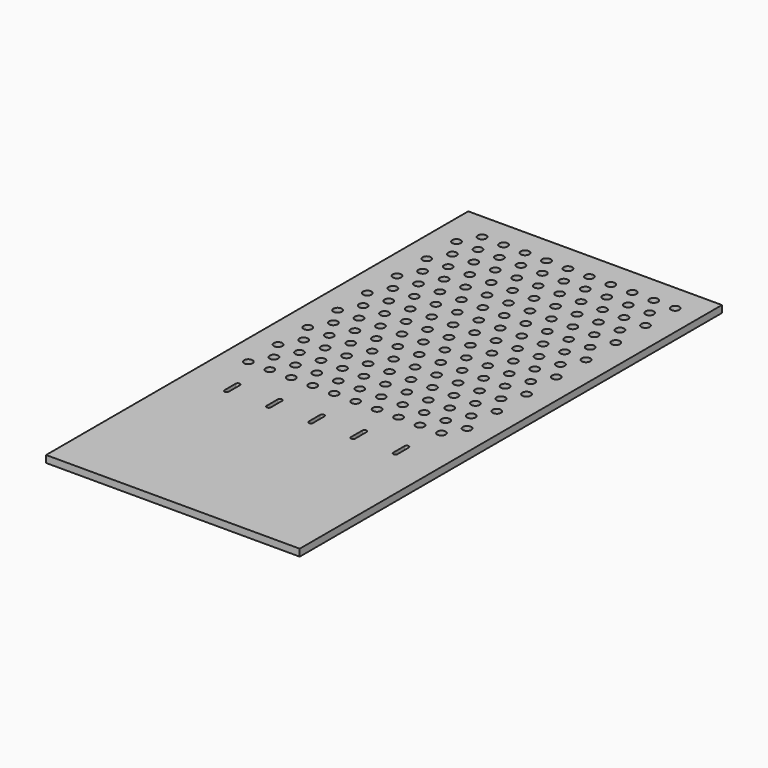
from build123d import *

# Parameters (mm, degrees)
F0_W     = 360.5
F0_H     = 750
F0_R     = 6
F1_DEPTH = 10
F3_DEPTH = 25


# Not quite as in the source:
# - a feature of the source that left no trace in its solid (it failed there, or was rolled back) is left out


with BuildPart() as f1:
    # F0 (on Top) → F1 (new body)
    with BuildSketch(Plane.XY):
        with Locations((145, 59.75)):
            Rectangle(F0_W, F0_H)
        Circle(F0_R, mode=Mode.SUBTRACT)
        with Locations((0, 52.828)):
            Circle(F0_R, mode=Mode.SUBTRACT)
        with Locations((30.5, 0)):
            Circle(F0_R, mode=Mode.SUBTRACT)
        with Locations((15.25, 26.4137748154)):
            Circle(F0_R, mode=Mode.SUBTRACT)
        with Locations((30.5, 52.828)):
            Circle(F0_R, mode=Mode.SUBTRACT)
        with Locations((45.75, 26.4137748154)):
            Circle(F0_R, mode=Mode.SUBTRACT)
        with Locations((61, 0)):
            Circle(F0_R, mode=Mode.SUBTRACT)
        with Locations((91.5, 0)):
            Circle(F0_R, mode=Mode.SUBTRACT)
        with Locations((76.25, 26.4137748154)):
            Circle(F0_R, mode=Mode.SUBTRACT)
        with Locations((61, 52.828)):
            Circle(F0_R, mode=Mode.SUBTRACT)
        with Locations((91.5, 52.828)):
            Circle(F0_R, mode=Mode.SUBTRACT)
        with Locations((122, 0)):
            Circle(F0_R, mode=Mode.SUBTRACT)
        with Locations((106.75, 26.4137748154)):
            Circle(F0_R, mode=Mode.SUBTRACT)
        with Locations((122, 52.828)):
            Circle(F0_R, mode=Mode.SUBTRACT)
        with Locations((137.25, 26.4137748154)):
            Circle(F0_R, mode=Mode.SUBTRACT)
        with Locations((152.5, 0)):
            Circle(F0_R, mode=Mode.SUBTRACT)
        with Locations((183, 0)):
            Circle(F0_R, mode=Mode.SUBTRACT)
        with Locations((152.5, 52.828)):
            Circle(F0_R, mode=Mode.SUBTRACT)
        with Locations((167.75, 26.4137748154)):
            Circle(F0_R, mode=Mode.SUBTRACT)
        with Locations((183, 52.828)):
            Circle(F0_R, mode=Mode.SUBTRACT)
        with Locations((213.5, 0)):
            Circle(F0_R, mode=Mode.SUBTRACT)
        with Locations((198.25, 26.4137748154)):
            Circle(F0_R, mode=Mode.SUBTRACT)
        with Locations((228.75, 26.4137748154)):
            Circle(F0_R, mode=Mode.SUBTRACT)
        with Locations((213.5, 52.828)):
            Circle(F0_R, mode=Mode.SUBTRACT)
        with Locations((244, 0)):
            Circle(F0_R, mode=Mode.SUBTRACT)
        with Locations((274.5, 0)):
            Circle(F0_R, mode=Mode.SUBTRACT)
        with Locations((244, 52.828)):
            Circle(F0_R, mode=Mode.SUBTRACT)
        with Locations((259.25, 26.4137748154)):
            Circle(F0_R, mode=Mode.SUBTRACT)
        with Locations((274.5, 52.828)):
            Circle(F0_R, mode=Mode.SUBTRACT)
        with Locations((289.75, 26.4137748154)):
            Circle(F0_R, mode=Mode.SUBTRACT)
        with Locations((0, 105.656)):
            Circle(F0_R, mode=Mode.SUBTRACT)
        with Locations((15.25, 79.2417748154)):
            Circle(F0_R, mode=Mode.SUBTRACT)
        with Locations((30.5, 105.656)):
            Circle(F0_R, mode=Mode.SUBTRACT)
        with Locations((45.75, 79.2417748154)):
            Circle(F0_R, mode=Mode.SUBTRACT)
        with Locations((15.25, 132.0697748154)):
            Circle(F0_R, mode=Mode.SUBTRACT)
        with Locations((45.75, 132.0697748154)):
            Circle(F0_R, mode=Mode.SUBTRACT)
        with Locations((0, 158.484)):
            Circle(F0_R, mode=Mode.SUBTRACT)
        with Locations((0, 211.312)):
            Circle(F0_R, mode=Mode.SUBTRACT)
        with Locations((30.5, 158.484)):
            Circle(F0_R, mode=Mode.SUBTRACT)
        with Locations((15.25, 184.8977748154)):
            Circle(F0_R, mode=Mode.SUBTRACT)
        with Locations((45.75, 184.8977748154)):
            Circle(F0_R, mode=Mode.SUBTRACT)
        with Locations((30.5, 211.312)):
            Circle(F0_R, mode=Mode.SUBTRACT)
        with Locations((15.25, 237.7257748154)):
            Circle(F0_R, mode=Mode.SUBTRACT)
        with Locations((45.75, 237.7257748154)):
            Circle(F0_R, mode=Mode.SUBTRACT)
        with Locations((76.25, 79.2417748154)):
            Circle(F0_R, mode=Mode.SUBTRACT)
        with Locations((61, 105.656)):
            Circle(F0_R, mode=Mode.SUBTRACT)
        with Locations((91.5, 105.656)):
            Circle(F0_R, mode=Mode.SUBTRACT)
        with Locations((76.25, 132.0697748154)):
            Circle(F0_R, mode=Mode.SUBTRACT)
        with Locations((106.75, 79.2417748154)):
            Circle(F0_R, mode=Mode.SUBTRACT)
        with Locations((122, 105.656)):
            Circle(F0_R, mode=Mode.SUBTRACT)
        with Locations((137.25, 79.2417748154)):
            Circle(F0_R, mode=Mode.SUBTRACT)
        with Locations((106.75, 132.0697748154)):
            Circle(F0_R, mode=Mode.SUBTRACT)
        with Locations((137.25, 132.0697748154)):
            Circle(F0_R, mode=Mode.SUBTRACT)
        with Locations((61, 158.484)):
            Circle(F0_R, mode=Mode.SUBTRACT)
        with Locations((76.25, 184.8977748154)):
            Circle(F0_R, mode=Mode.SUBTRACT)
        with Locations((91.5, 158.484)):
            Circle(F0_R, mode=Mode.SUBTRACT)
        with Locations((61, 211.312)):
            Circle(F0_R, mode=Mode.SUBTRACT)
        with Locations((76.25, 237.7257748154)):
            Circle(F0_R, mode=Mode.SUBTRACT)
        with Locations((91.5, 211.312)):
            Circle(F0_R, mode=Mode.SUBTRACT)
        with Locations((122, 158.484)):
            Circle(F0_R, mode=Mode.SUBTRACT)
        with Locations((106.75, 184.8977748154)):
            Circle(F0_R, mode=Mode.SUBTRACT)
        with Locations((137.25, 184.8977748154)):
            Circle(F0_R, mode=Mode.SUBTRACT)
        with Locations((122, 211.312)):
            Circle(F0_R, mode=Mode.SUBTRACT)
        with Locations((106.75, 237.7257748154)):
            Circle(F0_R, mode=Mode.SUBTRACT)
        with Locations((137.25, 237.7257748154)):
            Circle(F0_R, mode=Mode.SUBTRACT)
        with Locations((0, 264.14)):
            Circle(F0_R, mode=Mode.SUBTRACT)
        with Locations((0, 316.968)):
            Circle(F0_R, mode=Mode.SUBTRACT)
        with Locations((30.5, 264.14)):
            Circle(F0_R, mode=Mode.SUBTRACT)
        with Locations((15.25, 290.5537748154)):
            Circle(F0_R, mode=Mode.SUBTRACT)
        with Locations((45.75, 290.5537748154)):
            Circle(F0_R, mode=Mode.SUBTRACT)
        with Locations((30.5, 316.968)):
            Circle(F0_R, mode=Mode.SUBTRACT)
        with Locations((0, 369.796)):
            Circle(F0_R, mode=Mode.SUBTRACT)
        with Locations((15.25, 343.3817748154)):
            Circle(F0_R, mode=Mode.SUBTRACT)
        with Locations((30.5, 369.796)):
            Circle(F0_R, mode=Mode.SUBTRACT)
        with Locations((45.75, 343.3817748154)):
            Circle(F0_R, mode=Mode.SUBTRACT)
        with Locations((15.25, 396.2097748154)):
            Circle(F0_R, mode=Mode.SUBTRACT)
        with Locations((45.75, 396.2097748154)):
            Circle(F0_R, mode=Mode.SUBTRACT)
        with Locations((61, 264.14)):
            Circle(F0_R, mode=Mode.SUBTRACT)
        with Locations((76.25, 290.5537748154)):
            Circle(F0_R, mode=Mode.SUBTRACT)
        with Locations((91.5, 264.14)):
            Circle(F0_R, mode=Mode.SUBTRACT)
        with Locations((61, 316.968)):
            Circle(F0_R, mode=Mode.SUBTRACT)
        with Locations((91.5, 316.968)):
            Circle(F0_R, mode=Mode.SUBTRACT)
        with Locations((122, 264.14)):
            Circle(F0_R, mode=Mode.SUBTRACT)
        with Locations((106.75, 290.5537748154)):
            Circle(F0_R, mode=Mode.SUBTRACT)
        with Locations((137.25, 290.5537748154)):
            Circle(F0_R, mode=Mode.SUBTRACT)
        with Locations((122, 316.968)):
            Circle(F0_R, mode=Mode.SUBTRACT)
        with Locations((76.25, 343.3817748154)):
            Circle(F0_R, mode=Mode.SUBTRACT)
        with Locations((61, 369.796)):
            Circle(F0_R, mode=Mode.SUBTRACT)
        with Locations((91.5, 369.796)):
            Circle(F0_R, mode=Mode.SUBTRACT)
        with Locations((76.25, 396.2097748154)):
            Circle(F0_R, mode=Mode.SUBTRACT)
        with Locations((106.75, 343.3817748154)):
            Circle(F0_R, mode=Mode.SUBTRACT)
        with Locations((122, 369.796)):
            Circle(F0_R, mode=Mode.SUBTRACT)
        with Locations((137.25, 343.3817748154)):
            Circle(F0_R, mode=Mode.SUBTRACT)
        with Locations((106.75, 396.2097748154)):
            Circle(F0_R, mode=Mode.SUBTRACT)
        with Locations((137.25, 396.2097748154)):
            Circle(F0_R, mode=Mode.SUBTRACT)
        with Locations((152.5, 105.656)):
            Circle(F0_R, mode=Mode.SUBTRACT)
        with Locations((167.75, 79.2417748154)):
            Circle(F0_R, mode=Mode.SUBTRACT)
        with Locations((183, 105.656)):
            Circle(F0_R, mode=Mode.SUBTRACT)
        with Locations((167.75, 132.0697748154)):
            Circle(F0_R, mode=Mode.SUBTRACT)
        with Locations((198.25, 79.2417748154)):
            Circle(F0_R, mode=Mode.SUBTRACT)
        with Locations((228.75, 79.2417748154)):
            Circle(F0_R, mode=Mode.SUBTRACT)
        with Locations((213.5, 105.656)):
            Circle(F0_R, mode=Mode.SUBTRACT)
        with Locations((198.25, 132.0697748154)):
            Circle(F0_R, mode=Mode.SUBTRACT)
        with Locations((228.75, 132.0697748154)):
            Circle(F0_R, mode=Mode.SUBTRACT)
        with Locations((152.5, 158.484)):
            Circle(F0_R, mode=Mode.SUBTRACT)
        with Locations((183, 158.484)):
            Circle(F0_R, mode=Mode.SUBTRACT)
        with Locations((167.75, 184.8977748154)):
            Circle(F0_R, mode=Mode.SUBTRACT)
        with Locations((152.5, 211.312)):
            Circle(F0_R, mode=Mode.SUBTRACT)
        with Locations((183, 211.312)):
            Circle(F0_R, mode=Mode.SUBTRACT)
        with Locations((167.75, 237.7257748154)):
            Circle(F0_R, mode=Mode.SUBTRACT)
        with Locations((198.25, 184.8977748154)):
            Circle(F0_R, mode=Mode.SUBTRACT)
        with Locations((213.5, 158.484)):
            Circle(F0_R, mode=Mode.SUBTRACT)
        with Locations((228.75, 184.8977748154)):
            Circle(F0_R, mode=Mode.SUBTRACT)
        with Locations((198.25, 237.7257748154)):
            Circle(F0_R, mode=Mode.SUBTRACT)
        with Locations((213.5, 211.312)):
            Circle(F0_R, mode=Mode.SUBTRACT)
        with Locations((228.75, 237.7257748154)):
            Circle(F0_R, mode=Mode.SUBTRACT)
        with Locations((244, 105.656)):
            Circle(F0_R, mode=Mode.SUBTRACT)
        with Locations((259.25, 79.2417748154)):
            Circle(F0_R, mode=Mode.SUBTRACT)
        with Locations((274.5, 105.656)):
            Circle(F0_R, mode=Mode.SUBTRACT)
        with Locations((259.25, 132.0697748154)):
            Circle(F0_R, mode=Mode.SUBTRACT)
        with Locations((289.75, 79.2417748154)):
            Circle(F0_R, mode=Mode.SUBTRACT)
        with Locations((289.75, 132.0697748154)):
            Circle(F0_R, mode=Mode.SUBTRACT)
        with Locations((244, 158.484)):
            Circle(F0_R, mode=Mode.SUBTRACT)
        with Locations((274.5, 158.484)):
            Circle(F0_R, mode=Mode.SUBTRACT)
        with Locations((259.25, 184.8977748154)):
            Circle(F0_R, mode=Mode.SUBTRACT)
        with Locations((244, 211.312)):
            Circle(F0_R, mode=Mode.SUBTRACT)
        with Locations((274.5, 211.312)):
            Circle(F0_R, mode=Mode.SUBTRACT)
        with Locations((259.25, 237.7257748154)):
            Circle(F0_R, mode=Mode.SUBTRACT)
        with Locations((289.75, 184.8977748154)):
            Circle(F0_R, mode=Mode.SUBTRACT)
        with Locations((289.75, 237.7257748154)):
            Circle(F0_R, mode=Mode.SUBTRACT)
        with Locations((152.5, 264.14)):
            Circle(F0_R, mode=Mode.SUBTRACT)
        with Locations((183, 264.14)):
            Circle(F0_R, mode=Mode.SUBTRACT)
        with Locations((167.75, 290.5537748154)):
            Circle(F0_R, mode=Mode.SUBTRACT)
        with Locations((152.5, 316.968)):
            Circle(F0_R, mode=Mode.SUBTRACT)
        with Locations((183, 316.968)):
            Circle(F0_R, mode=Mode.SUBTRACT)
        with Locations((198.25, 290.5537748154)):
            Circle(F0_R, mode=Mode.SUBTRACT)
        with Locations((213.5, 264.14)):
            Circle(F0_R, mode=Mode.SUBTRACT)
        with Locations((228.75, 290.5537748154)):
            Circle(F0_R, mode=Mode.SUBTRACT)
        with Locations((213.5, 316.968)):
            Circle(F0_R, mode=Mode.SUBTRACT)
        with Locations((152.5, 369.796)):
            Circle(F0_R, mode=Mode.SUBTRACT)
        with Locations((167.75, 343.3817748154)):
            Circle(F0_R, mode=Mode.SUBTRACT)
        with Locations((183, 369.796)):
            Circle(F0_R, mode=Mode.SUBTRACT)
        with Locations((167.75, 396.2097748154)):
            Circle(F0_R, mode=Mode.SUBTRACT)
        with Locations((198.25, 343.3817748154)):
            Circle(F0_R, mode=Mode.SUBTRACT)
        with Locations((228.75, 343.3817748154)):
            Circle(F0_R, mode=Mode.SUBTRACT)
        with Locations((213.5, 369.796)):
            Circle(F0_R, mode=Mode.SUBTRACT)
        with Locations((198.25, 396.2097748154)):
            Circle(F0_R, mode=Mode.SUBTRACT)
        with Locations((228.75, 396.2097748154)):
            Circle(F0_R, mode=Mode.SUBTRACT)
        with Locations((244, 264.14)):
            Circle(F0_R, mode=Mode.SUBTRACT)
        with Locations((274.5, 264.14)):
            Circle(F0_R, mode=Mode.SUBTRACT)
        with Locations((259.25, 290.5537748154)):
            Circle(F0_R, mode=Mode.SUBTRACT)
        with Locations((244, 316.968)):
            Circle(F0_R, mode=Mode.SUBTRACT)
        with Locations((274.5, 316.968)):
            Circle(F0_R, mode=Mode.SUBTRACT)
        with Locations((289.75, 290.5537748154)):
            Circle(F0_R, mode=Mode.SUBTRACT)
        with Locations((244, 369.796)):
            Circle(F0_R, mode=Mode.SUBTRACT)
        with Locations((259.25, 343.3817748154)):
            Circle(F0_R, mode=Mode.SUBTRACT)
        with Locations((274.5, 369.796)):
            Circle(F0_R, mode=Mode.SUBTRACT)
        with Locations((259.25, 396.2097748154)):
            Circle(F0_R, mode=Mode.SUBTRACT)
        with Locations((289.75, 343.3817748154)):
            Circle(F0_R, mode=Mode.SUBTRACT)
        with Locations((289.75, 396.2097748154)):
            Circle(F0_R, mode=Mode.SUBTRACT)
    extrude(amount=F1_DEPTH)

    # F2 (on face) → F3 (cut)
    with BuildSketch(Plane.XY):
        with BuildLine():
            ThreePointArc((22, -50), (25, -53), (28, -50))
            ThreePointArc((28, -50), (25, -47), (22, -50))
        make_face()
        with BuildLine():
            ThreePointArc((82, -50), (85, -53), (88, -50))
            ThreePointArc((88, -50), (85, -47), (82, -50))
        make_face()
        with BuildLine():
            ThreePointArc((202, -50), (205, -53), (208, -50))
            ThreePointArc((208, -50), (205, -47), (202, -50))
        make_face()
        with BuildLine():
            ThreePointArc((142, -50), (145, -53), (148, -50))
            ThreePointArc((148, -50), (145, -47), (142, -50))
        make_face()
        with BuildLine():
            ThreePointArc((262, -50), (265, -53), (268, -50))
            ThreePointArc((268, -50), (265, -47), (262, -50))
        make_face()
        with BuildLine():
            Line((28, -70), (28, -50))
            ThreePointArc((28, -50), (25, -53), (22, -50))
            Line((22, -50), (22, -70))
            ThreePointArc((22, -70), (25, -67), (28, -70))
        make_face()
        with BuildLine():
            ThreePointArc((22, -70), (25, -73), (28, -70))
            ThreePointArc((28, -70), (25, -67), (22, -70))
        make_face()
        with BuildLine():
            Line((88, -70), (88, -50))
            ThreePointArc((88, -50), (85, -53), (82, -50))
            Line((82, -50), (82, -70))
            ThreePointArc((82, -70), (85, -67), (88, -70))
        make_face()
        with BuildLine():
            ThreePointArc((82, -70), (85, -73), (88, -70))
            ThreePointArc((88, -70), (85, -67), (82, -70))
        make_face()
        with BuildLine():
            ThreePointArc((142, -70), (145, -73), (148, -70))
            ThreePointArc((148, -70), (145, -67), (142, -70))
        make_face()
        with BuildLine():
            Line((148, -70), (148, -50))
            ThreePointArc((148, -50), (145, -53), (142, -50))
            Line((142, -50), (142, -70))
            ThreePointArc((142, -70), (145, -67), (148, -70))
        make_face()
        with BuildLine():
            ThreePointArc((202, -70), (205, -73), (208, -70))
            ThreePointArc((208, -70), (205, -67), (202, -70))
        make_face()
        with BuildLine():
            Line((208, -70), (208, -50))
            ThreePointArc((208, -50), (205, -53), (202, -50))
            Line((202, -50), (202, -70))
            ThreePointArc((202, -70), (205, -67), (208, -70))
        make_face()
        with BuildLine():
            Line((268, -70), (268, -50))
            ThreePointArc((268, -50), (265, -53), (262, -50))
            Line((262, -50), (262, -70))
            ThreePointArc((262, -70), (265, -67), (268, -70))
        make_face()
        with BuildLine():
            ThreePointArc((262, -70), (265, -73), (268, -70))
            ThreePointArc((268, -70), (265, -67), (262, -70))
        make_face()
    extrude(amount=F3_DEPTH, mode=Mode.SUBTRACT)


solid = f1.part
